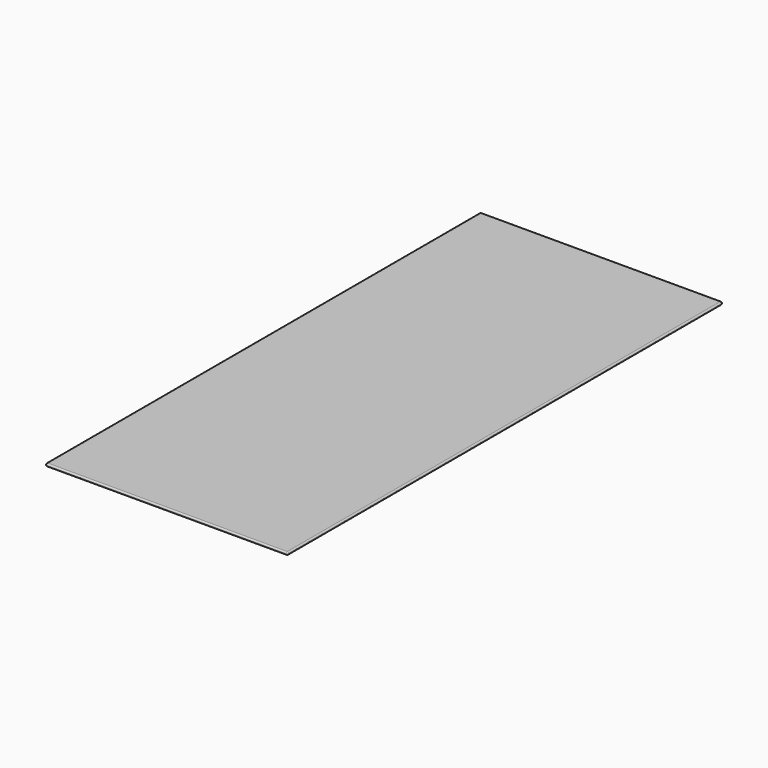
from build123d import *

# Parameters (mm, degrees)
F0_W     = 87.376
F0_H     = 196.2711086
F1_DEPTH = 1.016
F2_R     = 0.50799


# Not quite as in the source:
# - a fillet or chamfer is up to 0.001 mm smaller than in the source, because OpenCascade refuses the exact size


with BuildPart() as f1:
    # F0 (on Top) → F1 (new body)
    with BuildSketch(Plane.XY):
        Rectangle(F0_W, F0_H)
    extrude(amount=F1_DEPTH)

    # F2 (radius 0.508 in the source; OpenCascade refuses exactly that, so slightly less here)
    f2_edges = [f1.edges().sort_by_distance(p)[0] for p in [
        (43.688, 98.135554, 0.508),
        (-43.688, 98.135554, 0.508),
        (0, 98.135554, 0),
        (0, 98.135554, 1.016),
        (-43.688, -98.135554, 0.508),
        (-43.688, 0, 0),
        (-43.688, 0, 1.016),
        (43.688, -98.135554, 0.508),
        (0, -98.135554, 0),
        (0, -98.135554, 1.016),
        (43.688, 0, 0),
        (43.688, 0, 1.016),
    ]]
    fillet(f2_edges, radius=F2_R)


solid = f1.part
